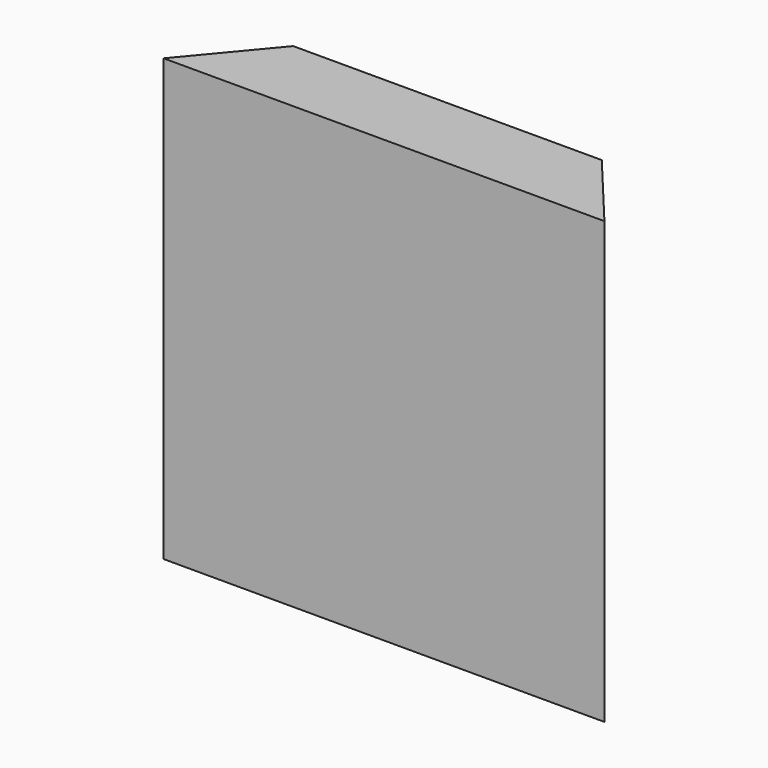
from build123d import *

# Parameters (mm, degrees)
F0_W       = 100
F0_H       = 100
F1_DEPTH   = 18
F2_SIZE2   = 14.99999
F2_SIZE    = 17.99999
F2_2_SIZE2 = 14.99999
F2_2_SIZE  = 17.99999
F3_R       = 2.5
F4_DEPTH   = 15


# Not quite as in the source:
# - a fillet or chamfer is up to 0.001 mm smaller than in the source, because OpenCascade refuses the exact size


with BuildPart() as f1:
    # F0 (on Front) → F1 (new body)
    with BuildSketch(Plane.XZ):
        Rectangle(F0_W, F0_H)
    extrude(amount=F1_DEPTH)

    # F2 (size 18 and 15 in the source; OpenCascade refuses exactly that, so slightly less here)
    f2_edges = [f1.edges().sort_by_distance(p)[0] for p in [
        (50, 0, 0),
    ]]
    f2_side = f1.faces().sort_by_distance((50, -9, 0))[0]
    chamfer(f2_edges, length=F2_SIZE, length2=F2_SIZE2, reference=f2_side)

    # F2#2 (size 18 and 15 in the source; OpenCascade refuses exactly that, so slightly less here)
    f2_2_edges = [f1.edges().sort_by_distance(p)[0] for p in [
        (-50, 0, 0),
    ]]
    f2_2_side = f1.faces().sort_by_distance((-50, -9, 0))[0]
    chamfer(f2_2_edges, length=F2_2_SIZE, length2=F2_2_SIZE2, reference=f2_2_side)

    # F3 (on face) → F4 (cut)
    with BuildSketch(Plane(origin=(0, 0, 0), x_dir=(-1, 0, 0), z_dir=(0, 1, 0))):
        with Locations((0, -15)):
            Circle(F3_R)
        with Locations((0, 41)):
            Circle(F3_R)
    extrude(amount=-F4_DEPTH, mode=Mode.SUBTRACT)


solid = f1.part
